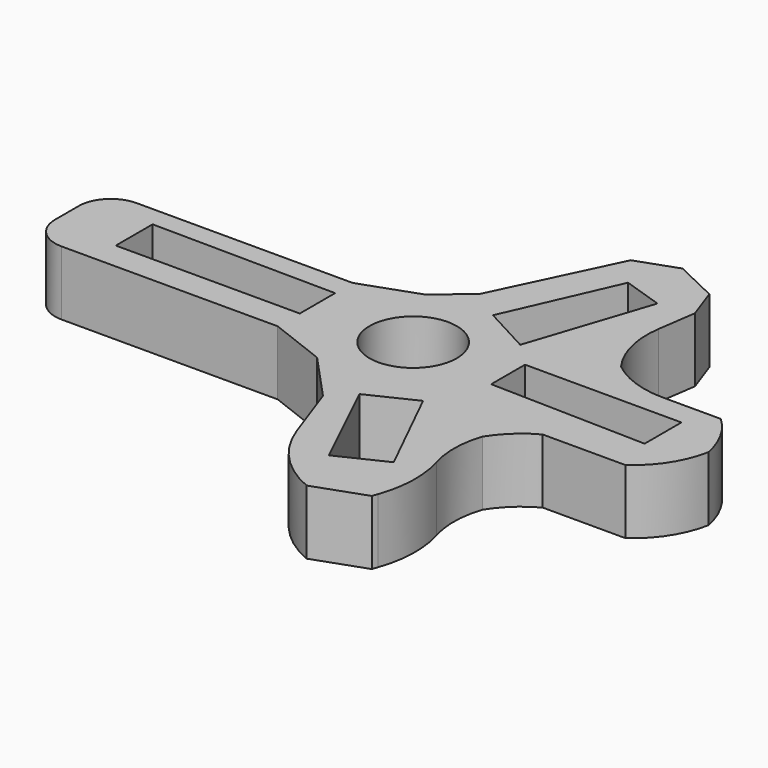
from build123d import *

# Parameters (mm, degrees)
F0_R        = 6.8863244876
F1_DEPTH    = 10.16
F2_T1_DEPTH = 66.6590982347
F2_T3_DEPTH = 42.201240443
F3_T1_DEPTH = 10.16
F3_T3_DEPTH = 58.4926144872
F3_T5_DEPTH = 51.6908183144
F4_R        = 5.08


# Not quite as in the source:
# - a fillet or chamfer that OpenCascade refuses, or shapes differently, is made with other operations: its cross-section is extruded or revolved along the edge and cut away or added


with BuildPart() as f1:
    # F0 (on Top) → F1 (new body)
    with BuildSketch(Plane.XY):
        Polygon((10.6026988985, 15.246915631), (5.517931655, 10.8906533569), (-3.485009307, 7.6960618608), (-42.6913611591, 7.6960618608), (-42.6913611591, -7.1152271703), (-3.485009307, -7.1152271703), (5.517931655, -10.6002362445), (12.4879479408, -18.1510895491), (19.5621072062, -38.0873594287), (25.8471500129, -38.0873594287), (33.8609059311, -35.2437690269), (36.3021790981, -28.315698728), (32.69538281, -18.1510895491), (36.3021790981, -10.6002362445), (40.0547920587, -9.2686640946), (53.1463883817, -9.2686640946), (59.2151660388, -7.1152271703), (59.2151660388, 5.3727226332), (54.5984730124, 7.6960618608), (40.0547920587, 7.6960618608), (36.3021790981, 10.8906533569), (32.69538281, 15.246915631), (34.4987809541, 27.7348645031), (32.69538281, 32.8171690926), (25.8471500129, 36.0883464863), (19.4785206028, 33.8285105681), align=None)
        Polygon((15.6825426966, -14.9564975873), (22.9429770261, -11.4714885131), (30.3544697336, -26.5248827454), (22.9429770261, -30.0823998534), align=None, mode=Mode.SUBTRACT)
        Polygon((-32.5267501175, -2.7589655947), (-32.5267501175, 4.501469899), (-3.485009307, 4.2110527866), (-3.485009307, -2.7589655947), align=None, mode=Mode.SUBTRACT)
        with Locations((12.1975308284, 0)):
            Circle(F0_R, mode=Mode.SUBTRACT)
        Polygon((51.4038838446, -3.339800518), (26.7184022814, -2.7589655947), (26.7184022814, 3.9206352085), (51.4038838446, 3.9206352085), align=None, mode=Mode.SUBTRACT)
        Polygon((22.9429770261, 7.6960618608), (15.3921246529, 11.7619056255), (22.962263142, 28.9465700275), (29.2712664114, 26.8636122346), align=None, mode=Mode.SUBTRACT)
    extrude(amount=F1_DEPTH)

    # F2: fillet of radius 18.1225687259 on 2 edges, made by hand

    # F2_s2 → F2_t1 (cut)
    with BuildSketch(Plane.XY.offset(-28.2495491174)):
        with BuildLine():
            ThreePointArc((15.7833367489, -27.4380957037), (19.6910161344, -33.825149661), (25.8471500129, -38.0873594287))
            Line((25.8471500129, -38.0873594287), (19.5621072062, -38.0873594287))
            Line((19.5621072062, -38.0873594287), (15.7833367489, -27.4380957037))
        make_face()
    extrude(amount=F2_T1_DEPTH, mode=Mode.SUBTRACT)

    # F2_s4 → F2_t3 (cut)
    with BuildSketch(Plane.XY.offset(-16.0206202215)):
        with BuildLine():
            ThreePointArc((34.1724327506, -34.3596894675), (35.202544115, -28.3169031391), (34.15919812, -22.2763878325))
            Line((34.15919812, -22.2763878325), (36.3021790981, -28.315698728))
            Line((36.3021790981, -28.315698728), (34.1724327506, -34.3596894675))
        make_face()
    extrude(amount=F2_T3_DEPTH, mode=Mode.SUBTRACT)

    # F3: fillet of radius 14.545063472 on 6 edges, made by hand

    # F3_s2 → F3_t1 (join)
    with BuildSketch(Plane.XY):
        with BuildLine():
            ThreePointArc((33.6130817468, 21.6016839559), (33.901548417, 15.9810300876), (36.3021790981, 10.8906533569))
            Line((36.3021790981, 10.8906533569), (32.69538281, 15.246915631))
            Line((32.69538281, 15.246915631), (33.6130817468, 21.6016839559))
        make_face()
        with BuildLine():
            ThreePointArc((36.3021790981, 10.8906533569), (40.5775055267, 8.5179295182), (45.3975437049, 7.6960618608))
            Line((45.3975437049, 7.6960618608), (40.0547920587, 7.6960618608))
            Line((40.0547920587, 7.6960618608), (36.3021790981, 10.8906533569))
        make_face()
        with BuildLine():
            ThreePointArc((35.2695823203, -12.7619848351), (33.8938078195, -17.8922695477), (34.4517445702, -23.1744360815))
            Line((34.4517445702, -23.1744360815), (33.0574978105, -23.5887604555))
            ThreePointArc((33.0574978105, -23.5887604555), (32.7884309604, -22.7627890129), (31.3246156504, -18.6374907295))
            Line((31.3246156504, -18.6374907295), (31.3829198252, -17.5241687984))
            Line((31.3829198252, -17.5241687984), (33.9571193355, -12.1350640844))
            Line((33.9571193355, -12.1350640844), (35.2695823203, -12.7619848351))
        make_face()
        with BuildLine():
            ThreePointArc((40.0547920587, -9.2686640946), (36.4117244984, -12.043489977), (33.8119770372, -15.8134917097))
            Line((33.8119770372, -15.8134917097), (36.3021790981, -10.6002362445))
            Line((36.3021790981, -10.6002362445), (40.0547920587, -9.2686640946))
        make_face()
    extrude(amount=F3_T1_DEPTH)

    # F3_s4 → F3_t3 (cut)
    with BuildSketch(Plane.XY.offset(-24.1663072436)):
        with BuildLine():
            ThreePointArc((59.2151660388, 2.5512957272), (57.6093256229, -4.0921505253), (53.1463883817, -9.2686640946))
            Line((53.1463883817, -9.2686640946), (59.2151660388, -7.1152271703))
            Line((59.2151660388, -7.1152271703), (59.2151660388, 2.5512957272))
        make_face()
    extrude(amount=F3_T3_DEPTH, mode=Mode.SUBTRACT)

    # F3_s6 → F3_t5 (cut)
    with BuildSketch(Plane.XY.offset(-20.7654091572)):
        with BuildLine():
            ThreePointArc((54.5984730124, 7.6960618608), (58.011160428, 2.8609568294), (59.2151660388, -2.9334410297))
            Line((59.2151660388, -2.9334410297), (59.2151660388, 5.3727226332))
            Line((59.2151660388, 5.3727226332), (54.5984730124, 7.6960618608))
        make_face()
    extrude(amount=F3_T5_DEPTH, mode=Mode.SUBTRACT)

    # F4
    f4_edges = [f1.edges().sort_by_distance(p)[0] for p in [
        (-42.691361, 7.696062, 5.08),
        (-42.691361, -7.115227, 5.08),
    ]]
    fillet(f4_edges, radius=F4_R)


solid = f1.part
